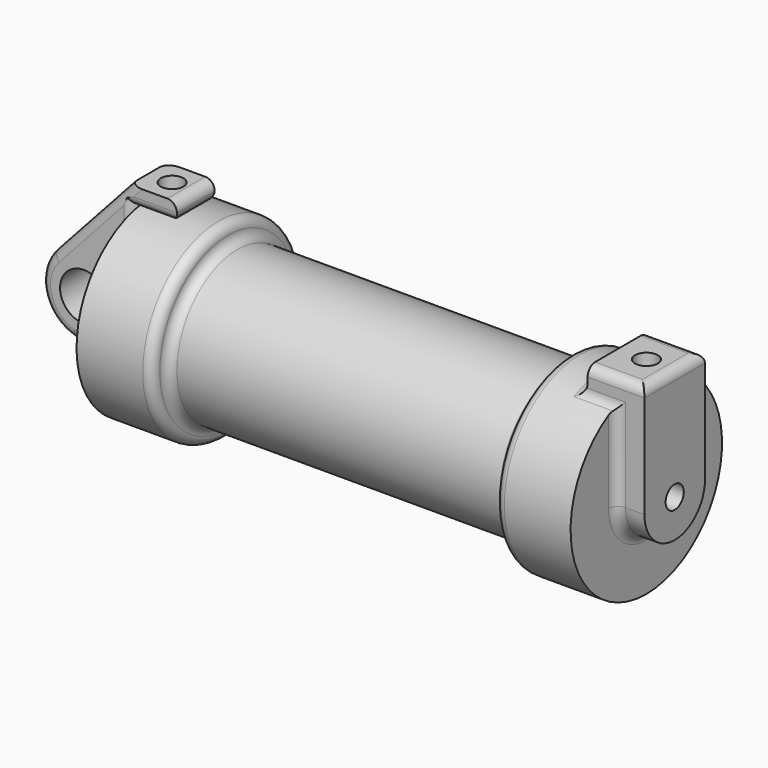
from build123d import *

# Parameters (mm, degrees)
F0_R          = 3.175
F1_DEPTH      = 3.175
F0_W          = 5.842
F0_H          = 12.7
F3_R          = 1.524
F4_DEPTH      = 3.81
F5_R          = 1.5247034047
F6_DEPTH      = 10.414
F7_R          = 1.5261104457
F8_DEPTH      = 17.78
F9_R          = 1.26999
F10_R         = 1.27
F11_T1_DEPTH  = 12.7
F11_T3_DEPTH  = 18.5821257943
F11_T5_DEPTH  = 12.7
F11_T7_DEPTH  = 9.017
F11_T9_DEPTH  = 17.7294216388
F11_T12_ANGLE = 116.8111069241
F11_T14_ANGLE = 116.8111069241
F11_T19_DEPTH = 15.875
F11_T23_DEPTH = 12.192
F11_T30_DEPTH = 15.875
F11_T34_DEPTH = 12.192
F12_R         = 1.27


# Not quite as in the source:
# - a fillet or chamfer that OpenCascade refuses, or shapes differently, is made with other operations: its cross-section is extruded or revolved along the edge and cut away or added
# - a fillet or chamfer is up to 0.001 mm smaller than in the source, because OpenCascade refuses the exact size


with BuildPart() as f1:
    # F0 (on Front) → F1 (new body, symmetric)
    with BuildSketch(Plane.XZ):
        with BuildLine():
            ThreePointArc((-8.1826630726, -5.5069827884), (-3.1957909266, -4.5493385486), (-0.9398, 0))
            ThreePointArc((-0.9398, 0), (-4.5919612295, 5.3297205562), (-10.8806298187, 3.8475430269))
            ThreePointArc((-10.8806298187, 3.8475430269), (-12.1459778134, -1.5837270034), (-8.1826630726, -5.5069827884))
        make_face()
        with Locations((-6.6548, 0)):
            Circle(F0_R, mode=Mode.SUBTRACT)
        with BuildLine():
            Line((-0.9398, 0), (0, 0))
            Line((0, 0), (0, 12.7))
            Line((0, 12.7), (5.842, 12.7))
            Line((5.842, 12.7), (5.842, 15.24))
            Line((5.842, 15.24), (-0.508, 15.24))
            Line((-0.508, 15.24), (-10.8806298187, 3.8475430269))
            ThreePointArc((-10.8806298187, 3.8475430269), (-4.5919612295, 5.3297205562), (-0.9398, 0))
        make_face()
        with BuildLine():
            Line((5.842, 0), (0, 0))
            Line((0, 0), (-0.9398, 0))
            ThreePointArc((-0.9398, 0), (-3.1957909266, -4.5493385486), (-8.1826630726, -5.5069827884))
            Line((-8.1826630726, -5.5069827884), (5.842, -9.398))
            Line((5.842, -9.398), (5.842, 0))
        make_face()
    extrude(amount=F1_DEPTH, both=True)


with BuildPart() as f2:
    # F0 (on Front) → F2 (revolve)
    with BuildSketch(Plane.XZ):
        with Locations((2.921, 6.35)):
            Rectangle(F0_W, F0_H)
        Polygon((5.842, 12.7), (5.842, 0), (66.294, 0), (66.294, 12.7), (56.134, 12.7), (56.134, 10.16), (10.16, 10.16), (10.16, 12.7), align=None)
    revolve(axis=Axis((33.147, 0, 0), (-1, 0, 0)))

    # F3 (on face) → F4 (join, symmetric)
    with BuildSketch(Plane.YZ.offset(66.294)):
        with BuildLine():
            ThreePointArc((-5.08, 0), (0, 5.08), (5.08, 0))
            Line((5.08, 0), (5.08, 11.6397422652))
            ThreePointArc((5.08, 11.6397422652), (0, 12.7), (-5.08, 11.6397422652))
            Line((-5.08, 11.6397422652), (-5.08, 0))
        make_face()
        with BuildLine():
            ThreePointArc((-5.08, 0), (0, -5.08), (5.08, 0))
            ThreePointArc((5.08, 0), (0, 5.08), (-5.08, 0))
        make_face()
        Circle(F3_R, mode=Mode.SUBTRACT)
        with BuildLine():
            ThreePointArc((-5.08, 11.6397422652), (0, 12.7), (5.08, 11.6397422652))
            Line((5.08, 11.6397422652), (5.08, 15.0270918384))
            Line((5.08, 15.0270918384), (-5.08, 15.0270918384))
            Line((-5.08, 15.0270918384), (-5.08, 11.6397422652))
        make_face()
    extrude(amount=F4_DEPTH, both=True)

    # F5 (on face) → F6 (cut)
    with BuildSketch(Plane.XY.offset(15.0270918384)):
        with Locations((66.3019493222, 0.0139107933)):
            Circle(F5_R)
    extrude(amount=-F6_DEPTH, mode=Mode.SUBTRACT)


with BuildPart() as f8_tool:
    # F7 (on face) → F8 (new body)
    with BuildSketch(Plane.XY.offset(15.24)):
        with Locations((2.667, 0)):
            Circle(F7_R)
    extrude(amount=-F8_DEPTH)


with BuildPart() as f1_1:
    add(f1.part)

    # F8: cut by f8_tool
    add(f8_tool.part, mode=Mode.SUBTRACT)

    # F11: fillet of radius 1.27 on 12 edges, made by hand

    # F11_s2 → F11_t1 (cut)
    with BuildSketch(Plane.XY):
        with BuildLine():
            ThreePointArc((0, -1.905), (-0.3719743879, -2.8030256121), (-1.27, -3.175))
            Line((-1.27, -3.175), (0, -3.175))
            Line((0, -3.175), (0, -1.905))
        make_face()
        with BuildLine():
            ThreePointArc((0, 1.905), (-0.3719743879, 2.8030256121), (-1.27, 3.175))
            Line((-1.27, 3.175), (0, 3.175))
            Line((0, 3.175), (0, 1.905))
        make_face()
    extrude(amount=F11_T1_DEPTH, mode=Mode.SUBTRACT)

    # F11_s4 → F11_t3 (cut)
    with BuildSketch(Plane(origin=(9.4938886236, 0, 10.4273187748), x_dir=(0, 1, 0), z_dir=(-0.6732358752, 0, -0.7394277898))):
        with BuildLine():
            ThreePointArc((-3.175, -9.3657440555), (-2.8030256121, -10.2637696676), (-1.905, -10.6357440555))
            Line((-1.905, -10.6357440555), (-3.175, -10.6357440555))
            Line((-3.175, -10.6357440555), (-3.175, -9.3657440555))
        make_face()
        with BuildLine():
            ThreePointArc((3.175, -9.3657440555), (2.8030256121, -10.2637696676), (1.905, -10.6357440555))
            Line((1.905, -10.6357440555), (3.175, -10.6357440555))
            Line((3.175, -10.6357440555), (3.175, -9.3657440555))
        make_face()
    extrude(amount=F11_T3_DEPTH, mode=Mode.SUBTRACT)

    # F11_s6 → F11_t5 (cut)
    with BuildSketch(Plane.XZ.offset(-6.35)):
        with BuildLine():
            ThreePointArc((5.842, 13.97), (5.4700256121, 14.8680256121), (4.572, 15.24))
            Line((4.572, 15.24), (5.842, 15.24))
            Line((5.842, 15.24), (5.842, 13.97))
        make_face()
        with BuildLine():
            ThreePointArc((4.572, 12.7), (5.4700256121, 13.0719743879), (5.842, 13.97))
            Line((5.842, 13.97), (5.842, 12.7))
            Line((5.842, 12.7), (4.572, 12.7))
        make_face()
    extrude(amount=F11_T5_DEPTH, mode=Mode.SUBTRACT)

    # F11_s8 → F11_t7 (cut)
    with BuildSketch(Plane.YZ):
        with BuildLine():
            ThreePointArc((-1.905, 12.7), (-2.8030256121, 13.0719743879), (-3.175, 13.97))
            Line((-3.175, 13.97), (-3.175, 12.7))
            Line((-3.175, 12.7), (-1.905, 12.7))
        make_face()
        with BuildLine():
            ThreePointArc((3.175, 13.97), (2.8030256121, 13.0719743879), (1.905, 12.7))
            Line((1.905, 12.7), (3.175, 12.7))
            Line((3.175, 12.7), (3.175, 13.97))
        make_face()
    extrude(amount=F11_T7_DEPTH, mode=Mode.SUBTRACT)

    # F11_s10 → F11_t9 (cut)
    with BuildSketch(Plane(origin=(-6.179167626, 0, 1.7143547379), x_dir=(0, 1, 0), z_dir=(0.9636015378, 0, -0.2673426199))):
        with BuildLine():
            ThreePointArc((-3.175, -6.2241116667), (-2.8030256121, -7.1221372788), (-1.905, -7.4941116667))
            Line((-1.905, -7.4941116667), (-3.175, -7.4941116667))
            Line((-3.175, -7.4941116667), (-3.175, -6.2241116667))
        make_face()
        with BuildLine():
            ThreePointArc((3.175, -6.2241116667), (2.8030256121, -7.1221372788), (1.905, -7.4941116667))
            Line((1.905, -7.4941116667), (3.175, -7.4941116667))
            Line((3.175, -7.4941116667), (3.175, -6.2241116667))
        make_face()
    extrude(amount=F11_T9_DEPTH, mode=Mode.SUBTRACT)

    # F11_s11 → F11_t12 (revolve, cut)
    with BuildSketch(Plane(origin=(-3.0162650989, 0, -3.3128214309), x_dir=(0, 1, 0), z_dir=(0.6732358752, 0, 0.7394277898))):
        with BuildLine():
            ThreePointArc((-3.175, 9.3657440555), (-2.8030256121, 10.2637696676), (-1.905, 10.6357440555))
            Line((-1.905, 10.6357440555), (-3.175, 10.6357440555))
            Line((-3.175, 10.6357440555), (-3.175, 9.3657440555))
        make_face()
    revolve(axis=Axis((-6.6548, -3.175, 0), (0, -1, 0)), revolution_arc=F11_T12_ANGLE, mode=Mode.SUBTRACT)

    # F11_s13 → F11_t14 (revolve, cut)
    with BuildSketch(Plane(origin=(-3.0162650989, 0, -3.3128214309), x_dir=(0, 1, 0), z_dir=(0.6732358752, 0, 0.7394277898))):
        with BuildLine():
            ThreePointArc((3.175, 9.3657440555), (2.8030256121, 10.2637696676), (1.905, 10.6357440555))
            Line((1.905, 10.6357440555), (3.175, 10.6357440555))
            Line((3.175, 10.6357440555), (3.175, 9.3657440555))
        make_face()
    revolve(axis=Axis((-6.6548, 3.175, 0), (0, -1, 0)), revolution_arc=F11_T14_ANGLE, mode=Mode.SUBTRACT)


with BuildPart() as f2_1:
    add(f2.part)

    # F8: cut by f8_tool
    add(f8_tool.part, mode=Mode.SUBTRACT)

    # F9 (radius 1.27 in the source; OpenCascade refuses exactly that, so slightly less here)
    f9_edges = [f2_1.edges().sort_by_distance(p)[0] for p in [
        (56.134, 0, -12.7),
        (56.134, 0, -10.16),
        (10.16, 0, -10.16),
        (33.147, 0, 10.16),
    ]]
    fillet(f9_edges, radius=F9_R)

    # F10
    f10_edges = [f2_1.edges().sort_by_distance(p)[0] for p in [
        (10.16, 0, -11.42999),
        (10.16, 0, -12.7),
        (10.531971, 0, 10.531971),
        (11.42999, 0, -10.16),
    ]]
    fillet(f10_edges, radius=F10_R)

    # F12
    f12_edges = [f2_1.edges().sort_by_distance(p)[0] for p in [
        (66.294, 5.08, 5.819871),
        (66.294, -5.08, 5.819871),
        (66.294, 0, -5.08),
        (62.484, 2.594732, 12.43211),
        (62.484, -2.594732, 12.43211),
        (64.389, 5.08, 11.639742),
        (64.389, -5.08, 11.639742),
        (66.294, 5.08, 15.027092),
        (70.104, 0, 15.027092),
        (66.294, -5.08, 15.027092),
    ]]
    fillet(f12_edges, radius=F12_R)


with BuildPart() as f11_tool17:
    # F11_s18 → F11_t19 (new body)
    with BuildSketch(Plane.XY):
        with BuildLine():
            ThreePointArc((0, -1.905), (-0.3719743879, -2.8030256121), (-1.27, -3.175))
            Line((-1.27, -3.175), (0, -3.175))
            Line((0, -3.175), (0, -1.905))
        make_face()
    extrude(amount=F11_T19_DEPTH)

    split(bisect_by=Plane.XY.offset(12.7), keep=Keep.TOP)


with BuildPart() as f11_tool21:
    # F11_s22 → F11_t23 (new body)
    with BuildSketch(Plane.YZ.offset(-3.175)):
        with BuildLine():
            ThreePointArc((-1.905, 12.7), (-2.8030256121, 13.0719743879), (-3.175, 13.97))
            Line((-3.175, 13.97), (-3.175, 12.7))
            Line((-3.175, 12.7), (-1.905, 12.7))
        make_face()
    extrude(amount=F11_T23_DEPTH)

    split(bisect_by=Plane.YZ, keep=Keep.BOTTOM)


with BuildPart() as f11_tool17_1:
    add(f11_tool17.part)

    # F11_t25: intersect F11_tool21
    add(f11_tool21.part, mode=Mode.INTERSECT)


with BuildPart() as f1_2:
    add(f1_1.part)

    # F11_t15: cut F11_tool17
    add(f11_tool17_1.part, mode=Mode.SUBTRACT)


with BuildPart() as f11_tool28:
    # F11_s29 → F11_t30 (new body)
    with BuildSketch(Plane.XY):
        with BuildLine():
            ThreePointArc((0, 1.905), (-0.3719743879, 2.8030256121), (-1.27, 3.175))
            Line((-1.27, 3.175), (0, 3.175))
            Line((0, 3.175), (0, 1.905))
        make_face()
    extrude(amount=F11_T30_DEPTH)

    split(bisect_by=Plane.XY.offset(12.7), keep=Keep.TOP)


with BuildPart() as f11_tool32:
    # F11_s33 → F11_t34 (new body)
    with BuildSketch(Plane.YZ.offset(-3.175)):
        with BuildLine():
            ThreePointArc((3.175, 13.97), (2.8030256121, 13.0719743879), (1.905, 12.7))
            Line((1.905, 12.7), (3.175, 12.7))
            Line((3.175, 12.7), (3.175, 13.97))
        make_face()
    extrude(amount=F11_T34_DEPTH)

    split(bisect_by=Plane.YZ, keep=Keep.BOTTOM)


with BuildPart() as f11_tool28_1:
    add(f11_tool28.part)

    # F11_t36: intersect F11_tool32
    add(f11_tool32.part, mode=Mode.INTERSECT)


with BuildPart() as f1_3:
    add(f1_2.part)

    # F11_t26: cut F11_tool28
    add(f11_tool28_1.part, mode=Mode.SUBTRACT)


solid = Compound([f2_1.part, f1_3.part])
